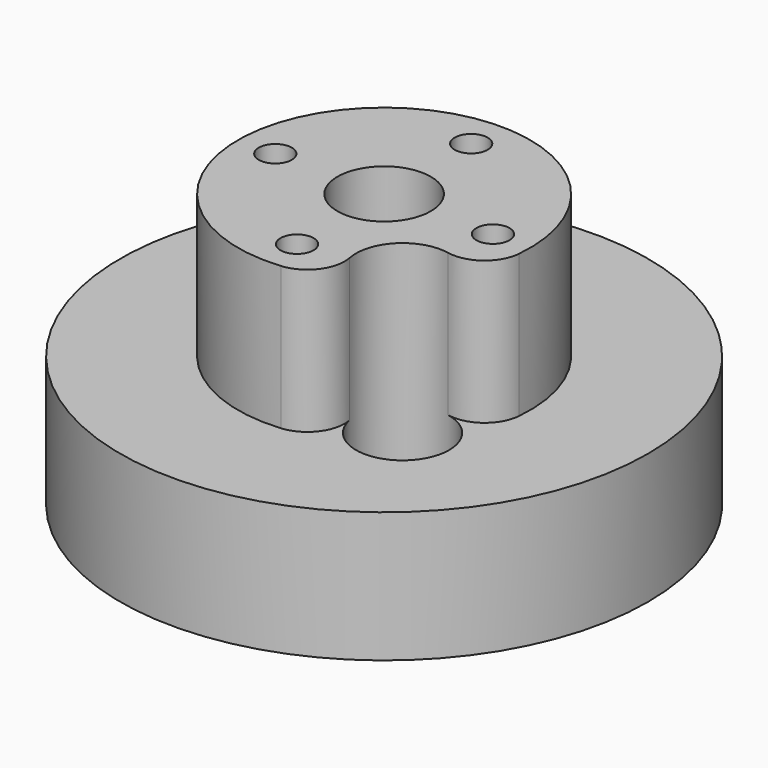
from build123d import *

# Parameters (mm, degrees)
F0_R     = 53.975
F1_DEPTH = 19.05
F2_R     = 29.87
F2_R_2   = 9.55
F3_DEPTH = 29.21
F5_D     = 6.7564
F6_R     = 53.975
F6_R_2   = 37.846
F7_DEPTH = 7.62
F8_R     = 9.525
F9_DEPTH = 55.881
F10_R    = 7.62


with BuildPart() as f1:
    # F0 (on Top) → F1 (new body)
    with BuildSketch(Plane.XY):
        Circle(F0_R)
    extrude(amount=F1_DEPTH)

    # F2 (on face) → F3 (join)
    with BuildSketch(Plane.XY.offset(19.05)):
        Circle(F2_R)
        Circle(F2_R_2, mode=Mode.SUBTRACT)
    extrude(amount=F3_DEPTH)

    # F5 (through all)
    with Locations(Plane.XY.offset(48.26)):
        with Locations((-22.25, 0), (0, 22.25), (22.25, 0), (0, -22.25)):
            Hole(F5_D / 2)

    # F6 (on face) → F7 (join)
    with BuildSketch(Plane(origin=(0, 0, 0), x_dir=(1, 0, 0), z_dir=(0, 0, -1))):
        Circle(F6_R)
        Circle(F6_R_2, mode=Mode.SUBTRACT)
    extrude(amount=F7_DEPTH)

    # F8 (on face) → F9 (cut, through all)
    with BuildSketch(Plane.XY.offset(48.26)):
        with Locations((18.8585378542, -18.8585378542)):
            Circle(F8_R)
    extrude(amount=-F9_DEPTH, mode=Mode.SUBTRACT)

    # F10
    f10_edges = [f1.edges().sort_by_distance(p)[0] for p in [
        (26.682506, -13.426122, 33.655),
        (13.426122, -26.682506, 33.655),
    ]]
    fillet(f10_edges, radius=F10_R)


solid = f1.part
